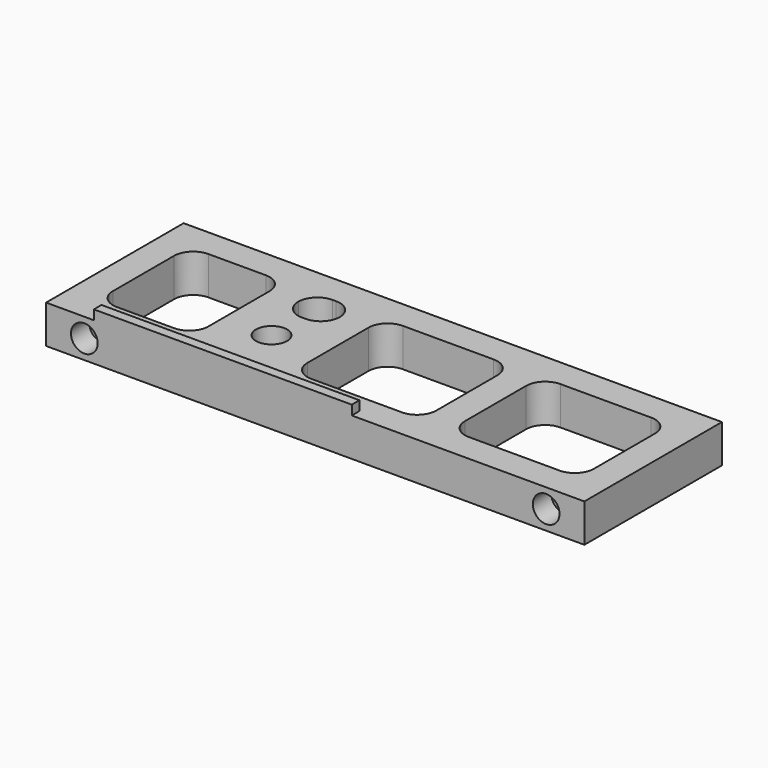
from build123d import *

# Parameters (mm, degrees)
F0_W      = 112.7
F0_H      = 36
F1_DEPTH  = 8
F3_W      = 54
F3_H      = 2
F4_DEPTH  = 2
F5_R      = 3.27
F6_DEPTH  = 8.001
F7_R      = 1.35
F8_DEPTH  = 5.5
F10_R     = 5.25
F11_DEPTH = 4.5
F9_W      = 20
F9_H      = 24
F9_W_2    = 27
F9_W_3    = 8.7
F9_H_2    = 8
F12_DEPTH = 10.001
F13_R     = 3.99999
F14_R     = 2.795
F15_DEPTH = 4.8
F16_R     = 2.795
F17_DEPTH = 4.8


# Not quite as in the source:
# - a fillet or chamfer is up to 0.001 mm smaller than in the source, because OpenCascade refuses the exact size


with BuildPart() as f1:
    # F0 (on Top) → F1 (new body)
    with BuildSketch(Plane.XY):
        Rectangle(F0_W, F0_H)
    extrude(amount=F1_DEPTH)

    # F3 (on face) → F4 (join)
    with BuildSketch(Plane.XY.offset(8)):
        with Locations((-19.35, -17)):
            Rectangle(F3_W, F3_H)
    extrude(amount=F4_DEPTH)

    # F5 (on face) → F6 (cut, through all)
    with BuildSketch(Plane.XY.offset(8)):
        with Locations((-20.35, -4)):
            Circle(F5_R)
    extrude(amount=-F6_DEPTH, mode=Mode.SUBTRACT)

    # F7 (on face) → F8 (cut)
    with BuildSketch(Plane(origin=(0, 0, 0), x_dir=(1, 0, 0), z_dir=(0, 0, -1))):
        with Locations((-53.85, 15)):
            Circle(F7_R)
        with Locations((-53.85, -15)):
            Circle(F7_R)
        with Locations((53.85, 15)):
            Circle(F7_R)
        with Locations((53.85, -15)):
            Circle(F7_R)
    extrude(amount=-F8_DEPTH, mode=Mode.SUBTRACT)

    # F10 (on face) → F11 (cut)
    with BuildSketch(Plane(origin=(0, 0, 0), x_dir=(1, 0, 0), z_dir=(0, 0, -1))):
        with Locations((-20.35, 4)):
            Circle(F10_R)
    extrude(amount=-F11_DEPTH, mode=Mode.SUBTRACT)

    # F9 (on face) → F12 (cut, through all)
    with BuildSketch(Plane(origin=(0, 0, 0), x_dir=(1, 0, 0), z_dir=(0, 0, -1))):
        with Locations((-40.35, 0)):
            Rectangle(F9_W, F9_H)
        with Locations((3.85, 0)):
            Rectangle(F9_W_2, F9_H)
        with Locations((36.85, 0)):
            Rectangle(F9_W_2, F9_H)
        with Locations((-20, -8)):
            Rectangle(F9_W_3, F9_H_2)
    extrude(amount=-F12_DEPTH, mode=Mode.SUBTRACT)

    # F13 (radius 4 in the source; OpenCascade refuses exactly that, so slightly less here)
    f13_edges = [f1.edges().sort_by_distance(p)[0] for p in [
        (-30.35, -12, 4),
        (-50.35, -12, 4),
        (-50.35, 12, 4),
        (-30.35, 12, 4),
        (-24.35, 4, 4),
        (-9.65, -12, 4),
        (23.35, -12, 4),
        (-9.65, 12, 4),
        (-24.35, 12, 4),
        (17.35, -12, 4),
        (50.35, -12, 4),
        (50.35, 12, 4),
        (23.35, 12, 4),
        (-15.65, 4, 4),
        (-15.65, 12, 4),
        (17.35, 12, 4),
    ]]
    fillet(f13_edges, radius=F13_R)

    # F14 (on face) → F15 (cut)
    with BuildSketch(Plane.XZ.offset(18)):
        with Locations((48.35, 4)):
            Circle(F14_R)
        with Locations((-48.35, 4)):
            Circle(F14_R)
    extrude(amount=-F15_DEPTH, mode=Mode.SUBTRACT)

    # F16 (on face) → F17 (cut)
    with BuildSketch(Plane(origin=(0, 18, 0), x_dir=(-1, 0, 0), z_dir=(0, 1, 0))):
        with Locations((48.35, 4)):
            Circle(F16_R)
        with Locations((-48.35, 4)):
            Circle(F16_R)
    extrude(amount=-F17_DEPTH, mode=Mode.SUBTRACT)


solid = f1.part
